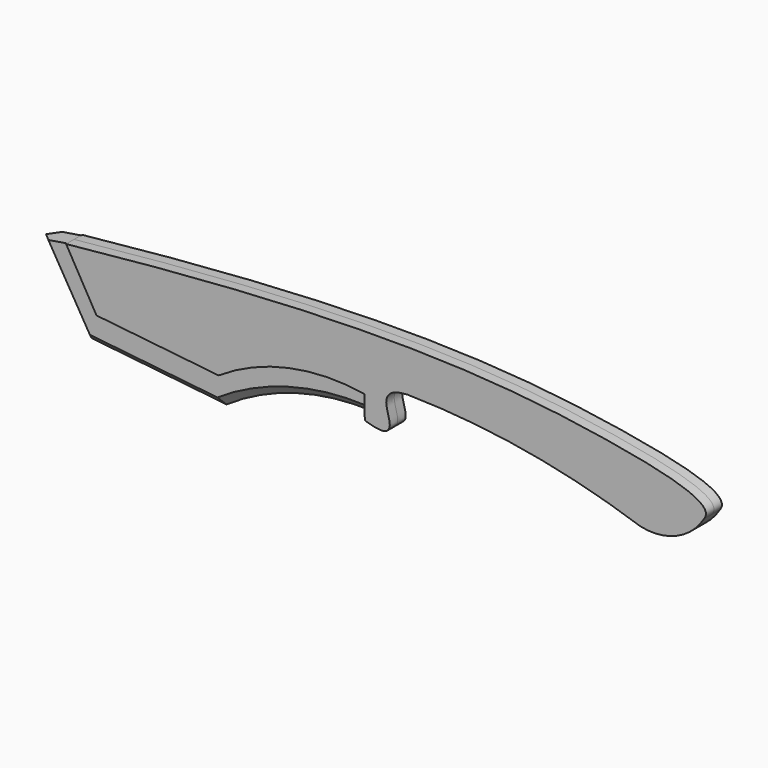
from build123d import *

# Parameters (mm, degrees)
F1_DEPTH = 2.032
F2_DEPTH = 1.778
F3_SIZE  = 1.77799
F4_R     = 5.08


# Not quite as in the source:
# - a fillet or chamfer is up to 0.001 mm smaller than in the source, because OpenCascade refuses the exact size


with BuildPart() as f1:
    # F0 (on Front) → F1 (new body, symmetric)
    with BuildSketch(Plane.XZ):
        with BuildLine():
            add(Edge.make_bspline(
                [(-62.7524927258, 28.1987972558), (-5.5860476855, 34.2682807977), (34.9384894232, 32.5216500899), (69.9510998155, 24.4512375904), (67.279830575, 21.1393777281)],
                knots=[0, 0, 0, 0, 0.7011346116, 1, 1, 1, 1], degree=3))
            Line((-62.7524927258, 28.1987972558), (-56.5566755831, 17.3903722316))
            Line((-56.5566755831, 17.3903722316), (-31.6641740501, 14.7209839443))
            ThreePointArc((-31.6641740501, 14.7209839443), (-17.3816327548, 20.703845911), (-1.9003116759, 21.0419595242))
            Line((-1.9003116759, 21.0419595242), (-1.9003116759, 17.1594452113))
            Line((-1.9003116759, 17.1594452113), (-1.7631361261, 16.3091998547))
            Line((-1.7631361261, 16.3091998547), (0, 15.8177418634))
            add(Edge.make_bspline(
                [(0, 15.8177418634), (1.0554286018, 15.6506710745), (2.4935673391, 15.483267377), (3.6762898855, 17.0941419119), (2.2318424188, 20.5970397753), (2.747819389, 22.4813980256), (4.3424194487, 23.5829041278), (5.8122159988, 23.7040893948), (6.7852635402, 23.7978529185)],
                knots=[0, 0, 0, 0, 0.1752354273, 0.3115686834, 0.5249745977, 0.6762943435, 0.8224611993, 1, 1, 1, 1], degree=3))
            ThreePointArc((6.7852635402, 23.7978529185), (30.8936565264, 21.5570594528), (54.3601624668, 15.5939338729))
            ThreePointArc((54.3601624668, 15.5939338729), (61.7117251, 16.2891237606), (67.279830575, 21.1393777281))
        make_face()
    extrude(amount=F1_DEPTH, both=True)


with BuildPart() as f2:
    # F0 (on Front) → F2 (new body, symmetric)
    with BuildSketch(Plane.XZ):
        Polygon((-56.5566755831, 17.3903722316), (-62.7524927258, 28.1987972558), (-68.4629157186, 27.2753052413), (-59.1897256672, 11.6384970024), align=None)
        Polygon((-31.6641740501, 14.7209839443), (-56.5566755831, 17.3903722316), (-59.1897256672, 11.6384970024), (-31.6641740501, 8.6867492646), align=None)
        with BuildLine():
            ThreePointArc((-1.9003116759, 21.0419595242), (-17.3816327548, 20.703845911), (-31.6641740501, 14.7209839443))
            Line((-31.6641740501, 14.7209839443), (-31.6641740501, 8.6867492646))
            ThreePointArc((-31.6641740501, 8.6867492646), (-17.4737066723, 15.3521509637), (-1.9003116759, 17.1594452113))
            Line((-1.9003116759, 17.1594452113), (-1.9003116759, 21.0419595242))
        make_face()
    extrude(amount=F2_DEPTH, both=True)

    # F3 (size 1.778 in the source; OpenCascade refuses exactly that, so slightly less here)
    f3_edges = [f2.edges().sort_by_distance(p)[0] for p in [
        (-17.473707, -1.778, 15.352151),
        (-17.473707, 1.778, 15.352151),
        (-45.42695, -1.778, 10.162623),
        (-45.42695, 1.778, 10.162623),
        (-63.826321, -1.778, 19.456901),
        (-63.826321, 1.778, 19.456901),
    ]]
    chamfer(f3_edges, length=F3_SIZE)

    # F4
    f4_edges = [f2.edges().sort_by_distance(p)[0] for p in [
        (-45.117862, 1.778, 11.917662),
    ]]
    fillet(f4_edges, radius=F4_R)


solid = Compound([f1.part, f2.part])
